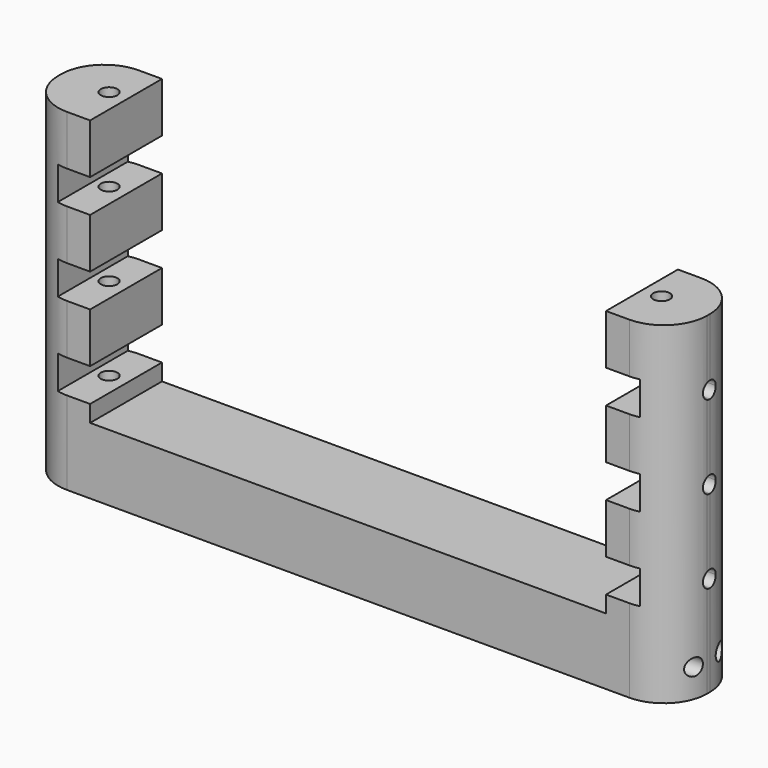
from build123d import *

# Parameters (mm, degrees)
F0_W         = 195
F0_H         = 100
F1_DEPTH     = 27
F2_W         = 155
F2_H         = 80
F3_DEPTH     = 27.001
F4_W         = 10
F4_H         = 10
F5_DEPTH     = 27.001
F6_R         = 2.5
F7_DEPTH     = 80
F9_DEPTH     = 195.001
F10_R        = 2.5
F11_DEPTH    = 195.001
F12_T1_DEPTH = 165


# Not quite as in the source:
# - a fillet or chamfer that OpenCascade refuses, or shapes differently, is made with other operations: its cross-section is extruded or revolved along the edge and cut away or added


with BuildPart() as f1:
    # F0 (on Front) → F1 (new body)
    with BuildSketch(Plane.XZ):
        with Locations((97.5, 50)):
            Rectangle(F0_W, F0_H)
    extrude(amount=F1_DEPTH)

    # F2 (on Front) → F3 (cut, through all)
    with BuildSketch(Plane.XZ):
        with Locations((97.5, 60)):
            Rectangle(F2_W, F2_H)
    extrude(amount=F3_DEPTH, mode=Mode.SUBTRACT)

    # F4 (on Front) → F5 (cut, through all)
    with BuildSketch(Plane.XZ):
        with Locations((180, 80)):
            Rectangle(F4_W, F4_H)
        with Locations((180, 55)):
            Rectangle(F4_W, F4_H)
        with Locations((180, 30)):
            Rectangle(F4_W, F4_H)
        with Locations((15, 30)):
            Rectangle(F4_W, F4_H)
        with Locations((15, 55)):
            Rectangle(F4_W, F4_H)
        with Locations((15, 80)):
            Rectangle(F4_W, F4_H)
    extrude(amount=F5_DEPTH, mode=Mode.SUBTRACT)

    # F6 (on face) → F7 (cut)
    with BuildSketch(Plane.XY.offset(100)):
        with Locations((180.5, -13)):
            Circle(F6_R)
        with Locations((14.5, -13)):
            Circle(F6_R)
    extrude(amount=-F7_DEPTH, mode=Mode.SUBTRACT)

    # F8 (on Right) → F9 (cut, through all)
    with BuildSketch(Plane.YZ):
        with BuildLine():
            Line((-13, 77.5), (-13, 82.5))
            ThreePointArc((-13, 82.5), (-15.5, 80), (-13, 77.5))
        make_face()
        with BuildLine():
            ThreePointArc((-13, 77.5), (-11.232233047, 78.232233047), (-10.5, 80))
            ThreePointArc((-10.5, 80), (-11.232233047, 81.767766953), (-13, 82.5))
            Line((-13, 82.5), (-13, 77.5))
        make_face()
        with BuildLine():
            Line((-13, 52.5), (-13, 57.5))
            ThreePointArc((-13, 57.5), (-15.5, 55), (-13, 52.5))
        make_face()
        with BuildLine():
            ThreePointArc((-10.5, 55), (-11.232233047, 56.767766953), (-13, 57.5))
            Line((-13, 57.5), (-13, 52.5))
            ThreePointArc((-13, 52.5), (-11.232233047, 53.232233047), (-10.5, 55))
        make_face()
        with BuildLine():
            Line((-13, 27.5), (-13, 32.5))
            ThreePointArc((-13, 32.5), (-15.5, 30), (-13, 27.5))
        make_face()
        with BuildLine():
            ThreePointArc((-10.5, 30), (-11.232233047, 31.767766953), (-13, 32.5))
            Line((-13, 32.5), (-13, 27.5))
            ThreePointArc((-13, 27.5), (-11.232233047, 28.232233047), (-10.5, 30))
        make_face()
    extrude(amount=F9_DEPTH, mode=Mode.SUBTRACT)

    # F10 (on Right) → F11 (cut, through all)
    with BuildSketch(Plane.YZ):
        with Locations((-8, 8.5)):
            Circle(F10_R)
        with Locations((-18, 8.5)):
            Circle(F10_R)
    extrude(amount=F11_DEPTH, mode=Mode.SUBTRACT)

    # F12: fillet of radius 13 on 4 edges, made by hand

    # F12_s2 → F12_t1 (cut)
    with BuildSketch(Plane.XY.offset(-32.5)):
        with BuildLine():
            ThreePointArc((0, -13), (3.8076118446, -3.8076118446), (13, 0))
            Line((13, 0), (0, 0))
            Line((0, 0), (0, -13))
        make_face()
        with BuildLine():
            ThreePointArc((0, -14), (3.8076118446, -23.1923881554), (13, -27))
            Line((13, -27), (0, -27))
            Line((0, -27), (0, -14))
        make_face()
        with BuildLine():
            ThreePointArc((182, -27), (191.1923881554, -23.1923881554), (195, -14))
            Line((195, -14), (195, -27))
            Line((195, -27), (182, -27))
        make_face()
        with BuildLine():
            ThreePointArc((182, 0), (191.1923881554, -3.8076118446), (195, -13))
            Line((195, -13), (195, 0))
            Line((195, 0), (182, 0))
        make_face()
    extrude(amount=F12_T1_DEPTH, mode=Mode.SUBTRACT)


solid = f1.part
